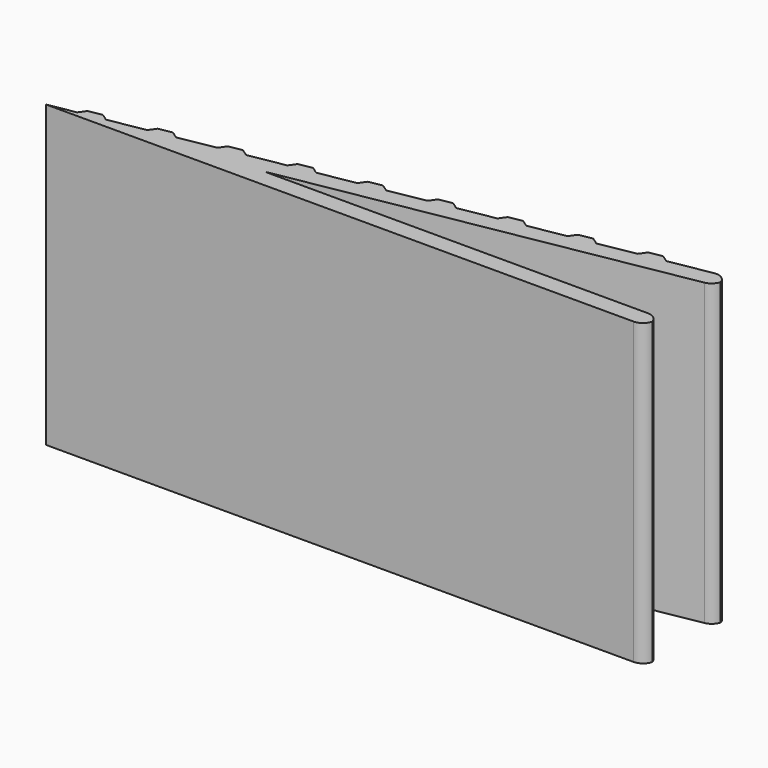
from build123d import *

# Parameters (mm, degrees)
F1_DEPTH    = 50
F2_T1_DEPTH = 61.9175359259
F2_T3_DEPTH = 58.3909963118
F2_T5_DEPTH = 60
F3_W        = 4.27056849
F3_H        = 50
F4_DEPTH    = 1
F5_SIZE     = 0.99999


# Not quite as in the source:
# - a fillet or chamfer that OpenCascade refuses, or shapes differently, is made with other operations: its cross-section is extruded or revolved along the edge and cut away or added
# - a fillet or chamfer is up to 0.001 mm smaller than in the source, because OpenCascade refuses the exact size


with BuildPart() as f1:
    # F0 (on Top) → F1 (new body)
    with BuildSketch(Plane.XY):
        Polygon((-53.1016754424, 0), (46.8983245576, 0), (46.8983245576, 3), (-19.0739845247, 3), (46.8983245576, 14.6326980708), (46.8983245576, 17.6326980708), align=None)
    extrude(amount=F1_DEPTH)

    # F2: fillet of radius 2 on 4 edges, made by hand

    # F2_s2 → F2_t1 (cut)
    with BuildSketch(Plane.XY.offset(-5.958767963)):
        with BuildLine():
            ThreePointArc((44.5510282023, 17.2188063917), (46.183899777, 16.7812797719), (46.8983245576, 15.2491908857))
            Line((46.8983245576, 15.2491908857), (46.8983245576, 17.6326980708))
            Line((46.8983245576, 17.6326980708), (44.5510282023, 17.2188063917))
        make_face()
    extrude(amount=F2_T1_DEPTH, mode=Mode.SUBTRACT)

    # F2_s4 → F2_t3 (cut)
    with BuildSketch(Plane.XY.offset(-4.1954981559)):
        with BuildLine():
            ThreePointArc((45.245620913, 14.3412818272), (46.4304134439, 15.0253221138), (46.8983245576, 16.3108973332))
            Line((46.8983245576, 16.3108973332), (46.8983245576, 14.6326980708))
            Line((46.8983245576, 14.6326980708), (45.245620913, 14.3412818272))
        make_face()
    extrude(amount=F2_T3_DEPTH, mode=Mode.SUBTRACT)

    # F2_s6 → F2_t5 (cut)
    with BuildSketch(Plane.XY.offset(-5)):
        with BuildLine():
            ThreePointArc((46.8983245576, 1), (46.31253812, 2.4142135624), (44.8983245576, 3))
            Line((44.8983245576, 3), (46.8983245576, 3))
            Line((46.8983245576, 3), (46.8983245576, 1))
        make_face()
        with BuildLine():
            ThreePointArc((44.8983245576, 0), (46.31253812, 0.5857864376), (46.8983245576, 2))
            Line((46.8983245576, 2), (46.8983245576, 0))
            Line((46.8983245576, 0), (44.8983245576, 0))
        make_face()
    extrude(amount=F2_T5_DEPTH, mode=Mode.SUBTRACT)

    # F3 (on face) → F4 (join)
    with BuildSketch(Plane(origin=(-1.6012114389, 9.0809213228, 0), x_dir=(-0.984807753, -0.1736481777, 0), z_dir=(-0.1736481777, 0.984807753, 0))):
        with Locations((45.5371029675, 25)):
            Rectangle(F3_W, F3_H)
        with Locations((35.1371029675, 25)):
            Rectangle(F3_W, F3_H)
        with Locations((24.7371029675, 25)):
            Rectangle(F3_W, F3_H)
        with Locations((14.3371029675, 25)):
            Rectangle(F3_W, F3_H)
        with Locations((3.9371029675, 25)):
            Rectangle(F3_W, F3_H)
        with Locations((-6.4628970325, 25)):
            Rectangle(F3_W, F3_H)
        with Locations((-16.8628970325, 25)):
            Rectangle(F3_W, F3_H)
        with Locations((-27.2628970325, 25)):
            Rectangle(F3_W, F3_H)
        with Locations((-37.6628970325, 25)):
            Rectangle(F3_W, F3_H)
    extrude(amount=F4_DEPTH)

    # F5 (size 1 in the source; OpenCascade refuses exactly that, so slightly less here)
    f5_edges = [f1.edges().sort_by_distance(p)[0] for p in [
        (-48.722996, 1.787506, 25),
        (-44.517307, 2.529082, 25),
        (-38.480996, 3.593447, 25),
        (-34.275307, 4.335023, 25),
        (-28.238995, 5.399388, 25),
        (-24.033306, 6.140964, 25),
        (-17.996994, 7.205329, 25),
        (-13.791305, 7.946905, 25),
        (-7.754994, 9.01127, 25),
        (-3.549305, 9.752847, 25),
        (2.487007, 10.817211, 25),
        (6.692696, 11.558788, 25),
        (12.729008, 12.623152, 25),
        (16.934697, 13.364729, 25),
        (22.971008, 14.429093, 25),
        (27.176697, 15.17067, 25),
        (33.213009, 16.235034, 25),
        (37.418698, 16.976611, 25),
    ]]
    chamfer(f5_edges, length=F5_SIZE)


solid = f1.part
